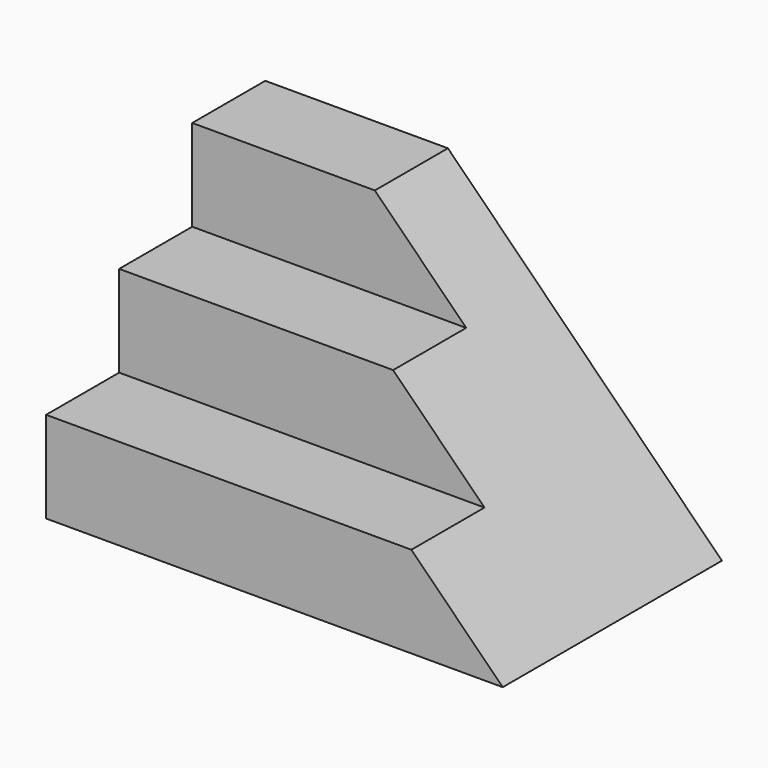
from build123d import *

# Parameters (mm, degrees)
F1_DEPTH    = 110
F2_T1_DEPTH = 380.0356183152


# Not quite as in the source:
# - a fillet or chamfer that OpenCascade refuses, or shapes differently, is made with other operations: its cross-section is extruded or revolved along the edge and cut away or added


with BuildPart() as f1:
    # F0 (on Right) → F1 (new body)
    with BuildSketch(Plane.YZ):
        Polygon((-60, 0), (0, 0), (0, 60), (-20, 60), (-20, 40), (-40, 40), (-40, 20), (-60, 20), align=None)
    extrude(amount=F1_DEPTH)

    # F2: chamfer of 70 on 1 edges, made by hand

    # F2_s2 → F2_t1 (cut)
    with BuildSketch(Plane.XZ.offset(-180.0178091576)):
        Polygon((40, 60), (110, -10), (110, 60), align=None)
    extrude(amount=F2_T1_DEPTH, mode=Mode.SUBTRACT)


solid = f1.part
